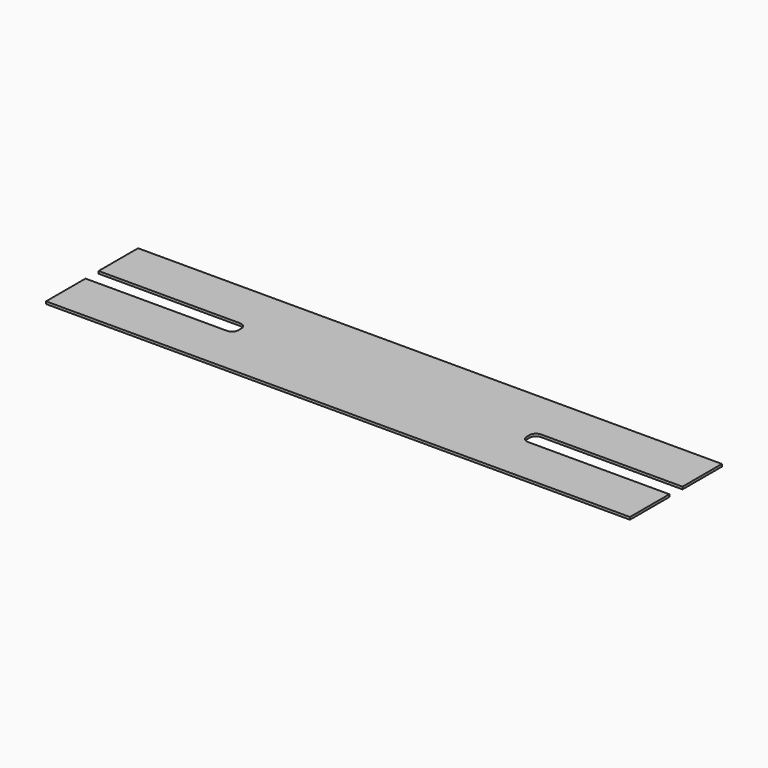
from build123d import *

# Parameters (mm, degrees)
F0_W     = 4
F0_H     = 3
F1_DEPTH = 0.15


# Not quite as in the source:
# - a feature names something its author has since deleted; it is built from what else it names


with BuildPart() as f1:
    # F0 (on Top) → F1 (new body)
    with BuildSketch(Plane.XY):
        with BuildLine():
            ThreePointArc((-8.775, -0.1), (-8.8921572875, -0.3828427125), (-9.175, -0.5))
            Line((-9.175, -0.5), (-13.775, -0.5))
            Line((-13.775, -0.5), (-13.775, -3.5))
            Line((-13.775, -3.5), (0, -3.5))
            Line((0, -3.5), (0, 3.5))
            Line((0, 3.5), (-13.775, 3.5))
            Line((-13.775, 3.5), (-13.775, 0.5))
            Line((-13.775, 0.5), (-9.175, 0.5))
            ThreePointArc((-9.175, 0.5), (-8.8921572875, 0.3828427125), (-8.775, 0.1))
            Line((-8.775, 0.1), (-8.775, -0.1))
        make_face()
        with Locations((-15.775, -2)):
            Rectangle(F0_W, F0_H)
        with BuildLine():
            Line((0, 3.5), (0, -3.5))
            Line((0, -3.5), (13.775, -3.5))
            Line((13.775, -3.5), (13.775, -0.5))
            Line((13.775, -0.5), (9.175, -0.5))
            ThreePointArc((9.175, -0.5), (8.8921572875, -0.3828427125), (8.775, -0.1))
            Line((8.775, -0.1), (8.775, 0.1))
            ThreePointArc((8.775, 0.1), (8.8921572875, 0.3828427125), (9.175, 0.5))
            Line((9.175, 0.5), (13.775, 0.5))
            Line((13.775, 0.5), (13.775, 3.5))
            Line((13.775, 3.5), (0, 3.5))
        make_face()
        with Locations((15.775, -2)):
            Rectangle(F0_W, F0_H)
        with Locations((-15.775, 2)):
            Rectangle(F0_W, F0_H)
        with Locations((15.775, 2)):
            Rectangle(F0_W, F0_H)
    extrude(amount=F1_DEPTH)


solid = f1.part
